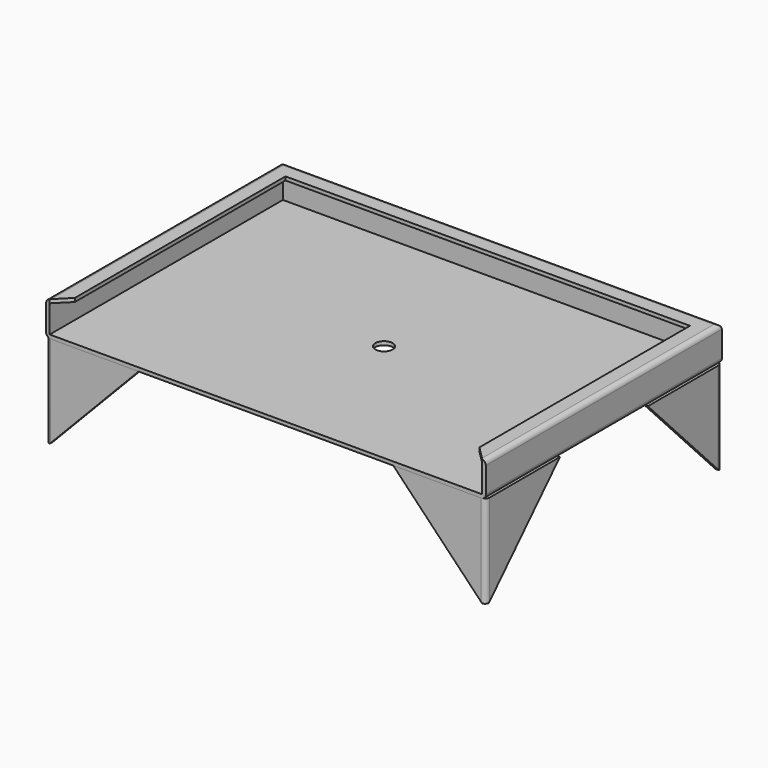
from build123d import *

# Parameters (mm, degrees)
F0_W      = 241.3
F0_H      = 161.925
F1_DEPTH  = 19.05
F3_T      = -1.984375
F4_W      = 221.9808846712
F4_H      = 152.4099913843
F5_DEPTH  = 5.17584
F7_DEPTH  = 50.8
F9_DEPTH  = 1.984375
F11_DEPTH = 1.984375
F14_R     = 2.54
F15_R     = 2.54
F15_2_R   = 2.54
F15_3_R   = 2.54
F15_4_R   = 2.54
F17_DEPTH = 1.984375
F19_D     = 9.525


# Not quite as in the source:
# - a length typed as a fraction of an inch, garbled in the dataset ("3 / 203.2 mm" for 3/8 in), is restored
# - a pattern or mirror of a feature is missing from the dataset's text; its kind, count and spacing are read off the source's solid


with BuildPart() as f1:
    # F0 (on Top) → F1 (new body)
    with BuildSketch(Plane.XY):
        Rectangle(F0_W, F0_H)
    extrude(amount=F1_DEPTH)

    # F3
    f3_openings = [f1.faces().sort_by_distance(p)[0] for p in [
        (0, -80.9625, 9.525),
    ]]
    offset(amount=F3_T, openings=f3_openings)

    # F4 (on face) → F5 (cut)
    with BuildSketch(Plane.XY.offset(19.05)):
        with Locations((0, -5.0618006591)):
            Rectangle(F4_W, F4_H)
    extrude(amount=-F5_DEPTH, mode=Mode.SUBTRACT)

    # F14
    f14_edges = [f1.edges().sort_by_distance(p)[0] for p in [
        (-120.65, 0, 19.05),
        (0, 80.9625, 19.05),
        (120.65, 0, 19.05),
        (-120.65, 0, 0),
        (0, 80.9625, 0),
        (120.65, 0, 0),
    ]]
    fillet(f14_edges, radius=F14_R)

    # F16 (on face) → F17 (cut, through all)
    with BuildSketch(Plane(origin=(0, 0, 17.065625), x_dir=(1, 0, 0), z_dir=(0, 0, -1))):
        Polygon((-110.9904423356, 73.2873173356), (-110.9904423356, 80.9625), (-118.665625, 80.9625), align=None)
    f17 = extrude(amount=-F17_DEPTH, mode=Mode.SUBTRACT)

    # F17_copies: F17 across plane
    add(f17.mirror(Plane(origin=(0, 0, 0), x_dir=(0, 0, 1), z_dir=(1, 0, 0))), mode=Mode.SUBTRACT)

    # F19 (through all)
    with Locations(Plane.XY.offset(19.05)):
        with Locations((0, 0)):
            Hole(F19_D / 2)


with BuildPart() as f7:
    # F6 (on face) → F7 (new body)
    with BuildSketch(Plane(origin=(0, 0, 0), x_dir=(1, 0, 0), z_dir=(0, 0, -1))):
        Polygon((-120.65, -80.9625), (-69.85, -80.9625), (-69.85, -78.978125), (-118.665625, -78.978125), (-118.665625, -30.1625), (-120.65, -30.1625), align=None)
    extrude(amount=F7_DEPTH)

    # F8 (on face) → F9 (cut, through all)
    with BuildSketch(Plane(origin=(-120.65, 0, 0), x_dir=(0, -1, 0), z_dir=(-1, 0, 0))):
        Polygon((-30.1625, 0), (-78.978125, -50.8), (-30.1625, -50.8), align=None)
    extrude(amount=-F9_DEPTH, mode=Mode.SUBTRACT)

    # F10 (on face) → F11 (cut, through all)
    with BuildSketch(Plane(origin=(0, 80.9625, 0), x_dir=(-1, 0, 0), z_dir=(0, 1, 0))):
        Polygon((118.665625, -50.8), (69.85, 0), (69.85, -50.8), align=None)
    extrude(amount=-F11_DEPTH, mode=Mode.SUBTRACT)


with BuildPart() as f12_1:
    # F12: instance of F7
    add(f7.part.mirror(Plane.YZ))


with BuildPart() as f13_1:
    # F13: instance of F12_1
    add(f12_1.part.mirror(Plane.XZ))

    # F15#3
    f15_3_edges = [f13_1.edges().sort_by_distance(p)[0] for p in [
        (120.65, -80.9625, -25.4),
    ]]
    fillet(f15_3_edges, radius=F15_3_R)


with BuildPart() as f13_2:
    # F13: instance of F7
    add(f7.part.mirror(Plane.XZ))

    # F15#4
    f15_4_edges = [f13_2.edges().sort_by_distance(p)[0] for p in [
        (-120.65, -80.9625, -25.4),
    ]]
    fillet(f15_4_edges, radius=F15_4_R)


with BuildPart() as f7_1:
    add(f7.part)

    # F15
    f15_edges = [f7_1.edges().sort_by_distance(p)[0] for p in [
        (-120.65, 80.9625, -25.4),
    ]]
    fillet(f15_edges, radius=F15_R)


with BuildPart() as f12_1_1:
    add(f12_1.part)

    # F15#2
    f15_2_edges = [f12_1_1.edges().sort_by_distance(p)[0] for p in [
        (120.65, 80.9625, -25.4),
    ]]
    fillet(f15_2_edges, radius=F15_2_R)


solid = Compound([f1.part, f13_1.part, f13_2.part, f7_1.part, f12_1_1.part])
